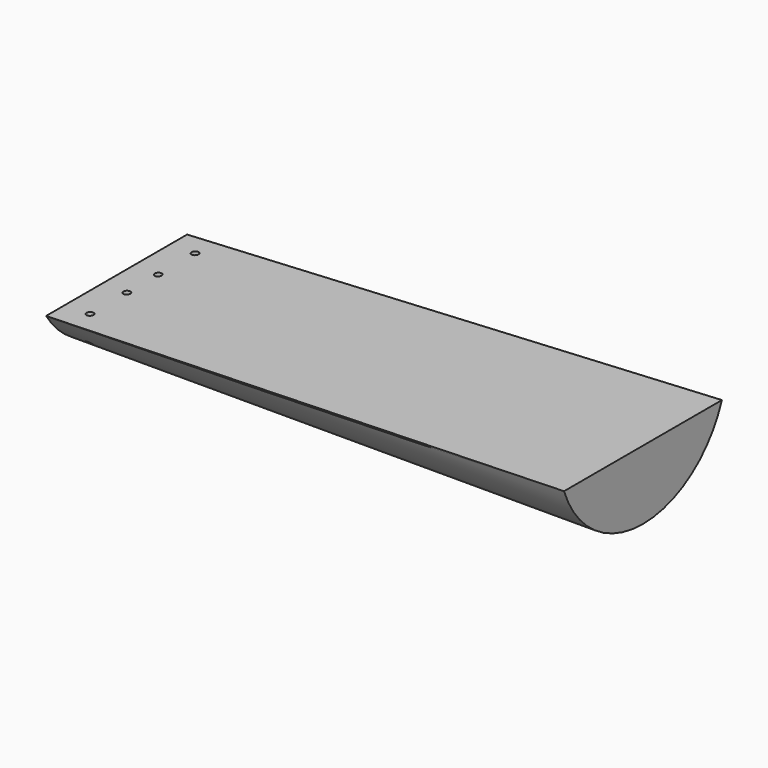
from build123d import *

# Parameters (mm, degrees)
F0_R          = 0.75
F1_DEPTH      = 14.986
F3_DEPTH      = 114.3
F5_DEPTH      = 25.4
F5_DEPTH_BACK = 25.4


# Not quite as in the source:
# - a feature names something its author has since deleted; it is built from what else it names


with BuildPart() as f1:
    # F0 (on Top) → F1 (new body)
    with BuildSketch(Plane.XY):
        Polygon((59.3341242821, 21.43125), (-59.3341242821, 19.05), (-59.3341242821, -19.05), (59.3341242821, -21.43125), align=None)
        with Locations((-49.3341242821, -14.2496579055)):
            Circle(F0_R, mode=Mode.SUBTRACT)
        with Locations((-49.3341242821, -4.2496579055)):
            Circle(F0_R, mode=Mode.SUBTRACT)
        with Locations((-49.3341242821, 4.2496579055)):
            Circle(F0_R, mode=Mode.SUBTRACT)
        with Locations((-49.3341242821, 14.2496579055)):
            Circle(F0_R, mode=Mode.SUBTRACT)
    extrude(amount=F1_DEPTH)

    # F2 (on face) → F3 (intersect)
    with BuildSketch(Plane.YZ.offset(59.3341242821)):
        with BuildLine():
            Line((21.43125, 14.986), (-21.43125, 14.986))
            ThreePointArc((-21.43125, 14.986), (-13.0755370179, 4.1181258353), (-1.54e-08, 0))
            ThreePointArc((-1.54e-08, 0), (13.0755370052, 4.1181258265), (21.43125, 14.986))
        make_face()
    extrude(amount=-F3_DEPTH, mode=Mode.INTERSECT)

    # F4 (on Front) → F5 (cut, two sides)
    with BuildSketch(Plane.XZ) as f5_sk:
        Polygon((-54.9658757179, 14.986), (-54.9658757179, 10.3923923096), (59.3341242821, 14.986), align=None)
    extrude(amount=-F5_DEPTH, mode=Mode.SUBTRACT)
    extrude(f5_sk.sketch, amount=F5_DEPTH_BACK, mode=Mode.SUBTRACT)


solid = f1.part
